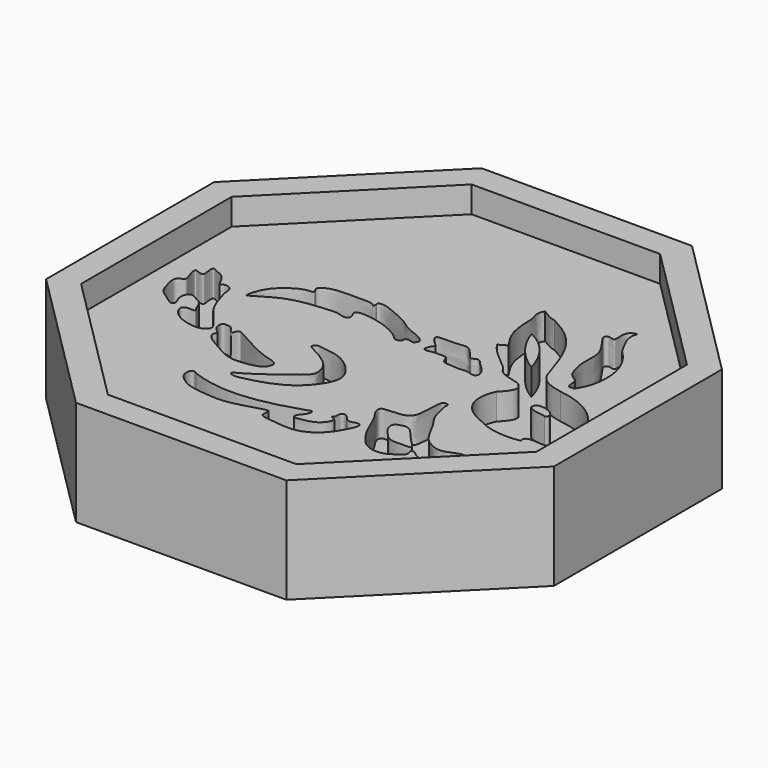
from build123d import *

# Parameters (mm, degrees)
F1_DEPTH = 25.4
F3_DEPTH = 6.35
F5_DEPTH = 6.35


with BuildPart() as f1:
    # F0 (on Top) → F1 (new body)
    with BuildSketch(Plane.XY):
        Polygon((-61.3372846899, 25.3607087968), (-61.3047391097, -25.4392807779), (-25.3607087968, -61.3372846899), (25.4392807779, -61.3047391097), (61.3372846899, -25.3607087968), (61.3047391097, 25.4392807779), (25.3607087968, 61.3372846899), (-25.4392807779, 61.3047391097), align=None)
    extrude(amount=F1_DEPTH)

    # F2 (on face) → F3 (cut)
    with BuildSketch(Plane.XY.offset(25.4)):
        Polygon((-54.9856008905, 22.734521413), (-54.9564255154, -22.8049569991), (-22.734521413, -54.9856008905), (22.8049569991, -54.9564255154), (54.9856008905, -22.734521413), (54.9564255154, 22.8049569991), (22.734521413, 54.9856008905), (-22.8049569991, 54.9564255154), align=None)
    extrude(amount=-F3_DEPTH, mode=Mode.SUBTRACT)

    # F4 (on face) → F5 (cut)
    with BuildSketch(Plane.XY.offset(19.05)):
        with BuildLine():
            add(Edge.make_bspline(
                [(12.8652052954, 32.6095893979), (14.2863783985, 31.7213572562), (15.3522584587, 31.0699865222), (16.5365692228, 30.8923404664)],
                knots=[0, 0, 0, 0, 4.0531292825, 4.0531292825, 4.0531292825, 4.0531292825], degree=3))
            add(Edge.make_bspline(
                [(12.8652052954, 32.6095893979), (11.5624647588, 31.0699865222), (12.8652052954, 29.569859306), (12.8652052954, 28.0499942601)],
                knots=[0, 0, 0, 0, 4.5595951378, 4.5595951378, 4.5595951378, 4.5595951378], degree=3))
            add(Edge.make_bspline(
                [(12.8652052954, 28.0499942601), (12.8652052954, 21.7139329761), (14.3455937505, 20.2335454524), (16.1220598966, 17.450414598)],
                knots=[0, 0, 0, 0, 11.0886514467, 11.0886514467, 11.0886514467, 11.0886514467], degree=3))
            add(Edge.make_bspline(
                [(16.1220598966, 17.450414598), (15.4904279237, 17.0951218655), (14.8587959508, 16.739829133), (14.2271639779, 16.3845364004)],
                knots=[0, 0, 0, 0, 2.1741036945, 2.1741036945, 2.1741036945, 2.1741036945], degree=3))
            add(Edge.make_bspline(
                [(14.2271639779, 16.3845364004), (16.4181385189, 12.7723887563), (20.6816550344, 10.9367063269), (21.8067504466, 8.5088703781)],
                knots=[0, 0, 0, 0, 10.930519033, 10.930519033, 10.930519033, 10.930519033], degree=3))
            add(Edge.make_bspline(
                [(21.8067504466, 8.5088703781), (23.6424319446, 6.8508354016), (27.4914409965, 6.9692670368), (27.6098717004, 5.9626027942)],
                knots=[0, 0, 0, 0, 6.3371677346, 6.3371677346, 6.3371677346, 6.3371677346], degree=3))
            add(Edge.make_bspline(
                [(27.6098717004, 5.9626027942), (28.7349671125, 5.3704483435), (28.9126131684, 3.9492752403), (26.1294841766, 1.2845764868)],
                knots=[0, 0, 0, 0, 4.9066768136, 4.9066768136, 4.9066768136, 4.9066768136], degree=3))
            add(Edge.make_bspline(
                [(26.1294841766, 1.2845764868), (23.7016472965, -4.3408987112), (26.3663455844, -7.9530458897), (31.2812328339, -9.8479427397)],
                knots=[0, 0, 0, 0, 12.2667639806, 12.2667639806, 12.2667639806, 12.2667639806], degree=3))
            add(Edge.make_bspline(
                [(31.2812328339, -9.8479427397), (35.0975431502, -11.920648627), (38.6735312641, -12.0461210608), (41.9044718146, -11.5755964071)],
                knots=[0, 0, 0, 0, 10.7628060299, 10.7628060299, 10.7628060299, 10.7628060299], degree=3))
            add(Edge.make_bspline(
                [(41.9044718146, -11.5755964071), (42.085633815, -11.5042446954), (42.4448295561, -11.3627733554), (41.9699487847, -10.9055818356), (42.4013458456, -10.2892093312), (42.9700330767, -9.9623558206), (44.339317482, -9.9303609692), (45.9999484886, -10.2190009461), (48.2650632898, -10.0226477297), (49.0421733777, -8.4974348176), (49.4673986841, -6.7818760612), (48.2356150706, -6.0112838819), (48.2111816709, -5.1344445173), (48.9546428188, -4.7180950966), (49.1552088222, -4.3385691075), (49.2499768734, -4.1592419147)],
                knots=[0, 0, 0, 0, 0.0517926528, 0.1026909632, 0.163872049, 0.2257582337, 0.3131365022, 0.4162991716, 0.5271779503, 0.6246107168, 0.7212866458, 0.8073521373, 0.8713533909, 0.939214083, 1, 1, 1, 1], degree=3))
            add(Edge.make_bspline(
                [(35.6039665639, 8.8641643524), (44.6259453893, 7.657723967), (49.1314120591, 2.2432615515), (49.2499768734, -4.1592419147)],
                knots=[0, 0, 0, 0, 18.8632634548, 18.8632634548, 18.8632634548, 18.8632634548], degree=3))
            add(Edge.make_bspline(
                [(29.0902592242, 13.4237594903), (29.9192778766, 10.0484741852), (33.2945622504, 9.3378880993), (35.6039665639, 8.8641643524)],
                knots=[0, 0, 0, 0, 7.9509930907, 7.9509930907, 7.9509930907, 7.9509930907], degree=3))
            add(Edge.make_bspline(
                [(16.5365692228, 30.8923404664), (24.7083120048, 26.7472546548), (26.1886995286, 22.1876576543), (29.0902592242, 13.4237594903)],
                knots=[0, 0, 0, 0, 21.5115423429, 21.5115423429, 21.5115423429, 21.5115423429], degree=3))
        make_face()
        with BuildLine():
            add(Edge.make_bspline(
                [(35.1602807641, 0.4698429548), (36.2895391881, -0.722153578), (38.6735312641, -0.5339434138), (39.4263714552, -0.8476267685)],
                knots=[0, 0, 0, 0, 4.4648915168, 4.4648915168, 4.4648915168, 4.4648915168], degree=3))
            add(Edge.make_bspline(
                [(35.1602807641, 0.4698429548), (35.003438592, 1.9127863925), (36.3522768021, 2.069628099), (37.8579571843, 1.6618396621)],
                knots=[0, 0, 0, 0, 2.9492904602, 2.9492904602, 2.9492904602, 2.9492904602], degree=3))
            add(Edge.make_bspline(
                [(37.8579571843, 1.6618396621), (40.5870005488, 0.8148947963), (40.3674244881, -1.0985733243), (39.4263714552, -0.8476267685)],
                knots=[0, 0, 0, 0, 2.9592811782, 2.9592811782, 2.9592811782, 2.9592811782], degree=3))
        make_face(mode=Mode.SUBTRACT)
        with BuildLine():
            add(Edge.make_bspline(
                [(16.5957845747, 23.8456930965), (17.7208781242, 20.1151147485), (20.8000857383, 15.6739503145), (25.0043887645, 13.2461134344)],
                knots=[0, 0, 0, 0, 13.5298083295, 13.5298083295, 13.5298083295, 13.5298083295], degree=3))
            add(Edge.make_bspline(
                [(16.5957845747, 23.8456930965), (21.1553797126, 21.7139348388), (23.8792933524, 17.6280625165), (25.0043887645, 13.2461134344)],
                knots=[0, 0, 0, 0, 13.5298083295, 13.5298083295, 13.5298083295, 13.5298083295], degree=3))
        make_face(mode=Mode.SUBTRACT)
        with BuildLine():
            add(Edge.make_bspline(
                [(36.7773883045, 11.3904932514), (36.5258197984, 11.4134308161), (36.0059714744, 11.441552121), (35.4683105712, 11.2022950388), (35.0849477198, 12.6846305445), (35.2044017719, 13.6366200305), (34.6569395769, 14.4413469981), (33.0252024985, 15.2566678667), (32.1524743097, 17.1164486402), (31.1629146199, 20.9798916279), (32.1715119956, 26.1591358134), (27.9018010841, 30.7101153681), (28.0217561467, 31.6738305022), (28.8396744959, 32.2666284081), (30.5133899031, 31.2777787574), (30.1501733126, 33.751637451), (30.3635645033, 35.1293956273), (31.0534006719, 35.9831194527), (32.5217684997, 36.4324470209), (31.9141483837, 35.4262952592), (31.9752447746, 33.6444442125), (32.6877917851, 32.0781371573), (33.7237389019, 29.9957571139), (34.2604020968, 29.1530700042), (34.501876682, 28.7738982588)],
                knots=[0, 0, 0, 0, 0.0319635023, 0.0550969569, 0.0962347495, 0.1325275562, 0.165994293, 0.2132001677, 0.2639019916, 0.3346772161, 0.4182092739, 0.5039036206, 0.5343069472, 0.567289738, 0.6075861256, 0.6559940549, 0.7003539611, 0.7383866916, 0.7752241506, 0.8051753553, 0.853499607, 0.9018762488, 0.9566720551, 1, 1, 1, 1], degree=3))
            add(Edge.make_bspline(
                [(36.7773883045, 11.3904932514), (39.463236928, 14.7851072252), (40.5450351536, 23.2529882342), (34.501876682, 28.7738982588)],
                knots=[0, 0, 0, 0, 17.5317062146, 17.5317062146, 17.5317062146, 17.5317062146], degree=3))
        make_face()
        with BuildLine():
            add(Edge.make_bspline(
                [(15.3017798439, 4.1850977577), (15.8504108693, 4.2177850474), (16.5550414794, 4.4887049852), (18.1896166173, 3.7142435012), (18.9757283165, 3.942597704), (19.4289979449, 4.7489757975), (18.5062489089, 6.7036354871), (16.5855031627, 8.1069206623), (15.8635662747, 9.3024818194), (14.8371871759, 9.4871226277), (14.006117554, 8.7324291205), (13.103768358, 9.4594760938), (12.3172770418, 10.6148024398), (10.7037012869, 12.421894333), (8.2663371615, 11.8028060837), (4.898617779, 11.9776625169), (2.8500336424, 11.7387445434), (4.0240421234, 10.0496599019), (4.8411169475, 9.3131721564), (5.6861925994, 8.7314147789), (4.8632757263, 7.994538167), (4.123946878, 5.7617188641), (7.0646114832, 6.6737619756), (9.4938960044, 6.3797840159), (10.0551516797, 6.4343790069), (10.5890638145, 4.3108599447), (12.1918688277, 4.4285767471), (14.4613292593, 4.1350239368), (15.3017798439, 4.1850977577)],
                knots=[0, 0, 0, 0, 0.0361277896, 0.0763539638, 0.1028571999, 0.1295711882, 0.1739091507, 0.2230620953, 0.2589689593, 0.2882258976, 0.3185345855, 0.3486027423, 0.3867925471, 0.4326179474, 0.4806856441, 0.5402453162, 0.5771081861, 0.6152551567, 0.6508315792, 0.6775455624, 0.7080799002, 0.7471334048, 0.7948687597, 0.8449259197, 0.8652135961, 0.9066525536, 0.9446556602, 1, 1, 1, 1], degree=3))
        make_face()
        with BuildLine():
            add(Edge.make_bspline(
                [(20.7343194634, -10.3275906295), (20.7709516831, -9.8598877606), (20.9158013429, -9.1476544453), (20.9635707176, -8.3262617691), (22.6524519262, -8.4637543763), (22.1858573154, -9.2863129669), (22.8103442257, -11.5488357773), (23.5016327468, -14.4918837995), (25.2439746955, -16.479295255), (26.7192648498, -19.6806321358), (28.4820205578, -22.3893117533), (30.5649842324, -23.6079937955), (32.7224685673, -24.3807567966), (35.2730051603, -23.378210488), (37.5654236583, -22.4783010118), (39.5446386208, -23.2424793874), (40.5050746182, -24.7881204138), (39.5650007167, -26.4962867217), (37.8128469366, -27.376918268), (35.2912661081, -28.2581182564), (33.3702752918, -28.9782017348), (30.9937489589, -29.088417311), (29.8397340381, -27.8310551705), (29.2156467184, -27.5106948573), (28.5387591084, -27.5359211724), (28.9890389277, -28.7818359483), (28.8075987021, -29.5377697234), (27.5485780868, -30.3867738592), (25.8135024785, -31.7677621319), (22.9716312634, -32.1429236281), (20.6399509233, -31.1555623423), (19.1403603495, -29.7183893954), (17.218559592, -26.9586403206), (16.1693959068, -24.4259222885), (14.8228571758, -21.2324016074), (13.1046488012, -19.1566371774), (13.2906663008, -17.6254241158), (14.4140267208, -17.4507651836), (16.5397677874, -17.2745262674), (18.8545261878, -17.2235756021), (20.4165119591, -15.7458789134), (20.4603473095, -14.0004061218), (20.7425460097, -12.1928979064), (20.6897030651, -10.8972317167), (20.7343194634, -10.3275906295)],
                knots=[0, 0, 0, 0, 0.0192942462, 0.0330741582, 0.052023046, 0.0651534831, 0.0913607937, 0.1216682951, 0.1495277699, 0.1820289015, 0.2130205143, 0.2394568776, 0.2648206079, 0.2930684248, 0.3200314682, 0.3440938321, 0.3657476976, 0.3880714073, 0.4123425116, 0.4405060774, 0.4657585875, 0.4915198065, 0.5133109298, 0.5277187881, 0.5387754002, 0.5568241908, 0.5717634667, 0.5922524986, 0.6181648002, 0.6469137153, 0.6737437891, 0.6986364849, 0.7298941842, 0.7590226893, 0.7913338923, 0.8195504419, 0.8381811992, 0.8549448831, 0.8804793546, 0.9068513478, 0.9306238126, 0.9529472238, 0.9765004747, 1, 1, 1, 1], degree=3))
        make_face()
        with BuildLine():
            add(Edge.make_bspline(
                [(22.8049569991, -26.4832917601), (21.7773803974, -26.1427349942), (20.7853597636, -24.7888072098), (19.4526932441, -23.4275348596), (19.0202822949, -21.3443208318), (20.4823026858, -20.6843131009), (22.5005362497, -20.2861010048), (24.4630261175, -22.5402330727), (26.0115860218, -24.4108868337), (27.5192963017, -25.7368526878), (27.8767415454, -26.6402760759), (27.0016791884, -26.6409491135), (24.1151934487, -26.917526918), (22.8049569991, -26.4832917601)],
                knots=[0, 0, 0, 0, 0.1074165587, 0.1986974636, 0.2853810353, 0.3613910674, 0.4510317064, 0.5602063852, 0.6661241164, 0.759241241, 0.8125419066, 0.8630359136, 1, 1, 1, 1], degree=3))
        make_face(mode=Mode.SUBTRACT)
        with BuildLine():
            add(Edge.make_bspline(
                [(-22.8500030935, -28.2156076282), (-23.1564221999, -28.0159332998), (-23.7152769634, -27.6517623089), (-24.3863424084, -28.1871627376), (-24.5625231079, -29.9486699359), (-23.3433241377, -31.3252949477), (-20.9932031236, -33.2067386928), (-15.22638086, -33.8351646845), (-10.1785100814, -34.0688360581), (-2.47913326, -31.1920867638), (-2.460426325, -32.046776882), (-2.3970225018, -32.8404748019), (-2.810640208, -34.2142542547), (2.0819787419, -34.5708039142), (6.7193859797, -35.1778319566), (11.7912536807, -32.1183129725), (14.0526674831, -27.6010297002), (14.5257017357, -26.4335554129), (14.6297205539, -25.2558639264), (13.4476452439, -25.0434674258), (12.677210255, -25.5824518196), (11.8921264481, -25.5053919057), (11.1659879121, -25.3350906316), (10.7521041426, -24.4270564162), (9.6833422485, -23.7478146611), (8.9110694031, -23.9254162985), (8.6366931415, -24.8331893315), (8.8904588509, -25.5996048999), (7.9621028526, -26.2811431455), (9.3608334823, -26.3303129622), (9.4999519076, -27.552032903), (7.796632177, -29.9619376165), (4.804334332, -30.4744649523), (3.3250515889, -30.808696151), (2.4506336317, -30.5166183135), (2.6073700045, -29.6227983207), (3.5136911361, -28.6934956319), (4.0114212731, -27.9436231109), (4.2838183347, -26.8876544187), (3.8082859259, -26.5723866906), (3.3697701718, -26.7870327785), (3.1157024205, -26.9113946706)],
                knots=[0, 0, 0, 0, 0.0200132257, 0.0365006172, 0.0622847867, 0.0892370717, 0.124007682, 0.1718500922, 0.2222414582, 0.2769290002, 0.2891044901, 0.3077607047, 0.3273219132, 0.3688671667, 0.4147463647, 0.4634655653, 0.5085506795, 0.5315635247, 0.5511247333, 0.5709731652, 0.5906705705, 0.6084161703, 0.6252452309, 0.6452755692, 0.6677696463, 0.6843028154, 0.7030430888, 0.721261059, 0.7378696831, 0.75676453, 0.7765156316, 0.8105318006, 0.8462195329, 0.8714235324, 0.888436846, 0.9057622096, 0.9290789036, 0.9493112706, 0.9693926854, 0.9822666996, 1, 1, 1, 1], degree=3))
            add(Edge.make_bspline(
                [(3.1157024205, -26.9113946706), (-6.5275733359, -30.1126465201), (-14.4714191556, -31.4168594778), (-22.8500030935, -28.2156076282)],
                knots=[0, 0, 0, 0, 25.9984390738, 25.9984390738, 25.9984390738, 25.9984390738], degree=3))
        make_face()
        with BuildLine():
            add(Edge.make_bspline(
                [(-10.6559619308, -5.2117551677), (-11.1737401757, -5.1362324872), (-11.7424506379, -4.9714464397), (-12.648442391, -5.4144357157), (-12.7500393741, -6.1161411911), (-12.3125446671, -6.4565452867), (-10.9405308104, -7.0731225678), (-9.1369698619, -8.0823065363), (-6.0712570972, -10.2151958876), (-5.2217867694, -12.6447334736), (-4.9746455567, -14.6813205825), (-7.5588855144, -16.9055478606), (-10.6532169743, -19.0485081325), (-14.4504219336, -22.0939945512), (-17.455448897, -23.5012935564), (-17.9230491301, -24.1027794323), (-16.6706066398, -24.7404310598), (-13.7255998954, -24.156814816), (-5.3862465252, -21.8767233991), (0.0120330444, -15.0338509057), (-0.1770248658, -10.6283446412), (-5.2708543932, -5.5843953024), (-9.5773732915, -5.3690771603), (-10.6559619308, -5.2117551677)],
                knots=[0, 0, 0, 0, 0.0310574833, 0.0576453165, 0.0794112577, 0.0992654413, 0.1335769874, 0.1762031417, 0.2313178012, 0.276910693, 0.3154710571, 0.3660978136, 0.4233404628, 0.4884366707, 0.5399210219, 0.5589256006, 0.5872706354, 0.636270169, 0.7212275866, 0.803887594, 0.8604004895, 0.9353038701, 1, 1, 1, 1], degree=3))
        make_face()
        with BuildLine():
            add(Edge.make_bspline(
                [(-22.2946368158, -19.1632434726), (-21.0493988148, -19.5119202164), (-18.6880382006, -19.4450553681), (-15.5481418092, -18.8919910447), (-14.0332293864, -17.8840870443), (-13.4955697372, -16.3469941527), (-14.1341895958, -15.4339327932), (-16.3883421895, -14.9050941461), (-19.8490922568, -13.5739760108), (-22.5931502921, -11.9756349915), (-26.078519987, -10.2568666189), (-26.8991210249, -9.5874929089), (-27.6901522691, -10.13266369), (-27.6203290749, -11.0788339927), (-28.6319524294, -10.7883304604), (-29.308762912, -9.2806269758), (-30.2719479537, -9.3408028948), (-31.8815711607, -8.945568532), (-31.7053750515, -11.3414838731), (-30.60133097, -12.272673542), (-29.7599805353, -12.7489968005), (-30.6848565625, -13.6607693821), (-29.5836041778, -15.4675565989), (-26.3586662834, -17.1279574729), (-23.6842152669, -18.7741502316), (-22.2946368158, -19.1632434726)],
                knots=[0, 0, 0, 0, 0.0622592495, 0.1194842442, 0.1621790015, 0.2007002522, 0.2312415619, 0.2794627383, 0.3419096516, 0.4020814388, 0.4652367387, 0.4959773841, 0.5239430148, 0.5511816552, 0.578209774, 0.6183631416, 0.649465769, 0.6848743271, 0.7281984959, 0.7682926938, 0.7951052662, 0.8255927665, 0.8680347902, 0.9305240353, 1, 1, 1, 1], degree=3))
        make_face()
        with BuildLine():
            add(Edge.make_bspline(
                [(-48.536233604, 0.5818881327), (-48.7993935081, 0.214424348), (-50.6232341136, -0.1406925801), (-49.5900537739, -3.567871753), (-48.9612726452, -6.0753250269), (-45.8419759594, -7.8890615195), (-44.5461860731, -8.9553314596), (-43.668018572, -8.2975634323), (-44.3455154017, -7.0124013614), (-44.7212608191, -5.7619723643), (-44.5464307201, -4.3277114714), (-43.475906841, -3.4658299441), (-41.9919242331, -4.3530284656), (-40.0910014917, -5.3334169649), (-39.7171833038, -7.116003175), (-38.6376000967, -8.4834991304), (-40.0099629337, -8.3881716907), (-41.220260459, -8.31457224), (-41.9367437761, -9.1059292531), (-41.7226121814, -9.6941307646), (-41.4943253777, -10.5163335894), (-39.6311525311, -12.4424849476), (-36.8731140753, -13.275454031), (-34.5043187855, -13.6223348002), (-32.8528768601, -13.1099659491), (-31.946682489, -12.1411358408), (-32.4510768522, -10.7397642295), (-34.6480914317, -8.2150297923), (-36.3991290059, -6.2732019618), (-37.8806992705, -3.4304789411), (-38.7339927463, -0.5836219813), (-39.1752539851, 1.0003629302), (-39.0635096274, 2.2340517971), (-40.1593292268, 3.6055012549), (-41.8496236937, 3.2097039443), (-41.8184773397, 2.3568461735), (-42.9403272041, 4.6014895605), (-44.0708022394, 6.1878150156), (-45.8347779568, 6.6928819631), (-47.3484563418, 7.7686503404), (-47.0497576663, 5.1475346558), (-46.7874060186, 3.9082822982), (-48.2830523519, 4.2933827218), (-49.6768094639, 4.9815397707), (-48.8456887547, 2.2143254407), (-48.2702506616, 0.9532938716), (-48.536233604, 0.5818881327)],
                knots=[0, 0, 0, 0, 0.0232700879, 0.0539157394, 0.0832957416, 0.1165416169, 0.138415086, 0.1530447808, 0.1731834999, 0.1941072535, 0.214856042, 0.2333825675, 0.2557602784, 0.2813606968, 0.3057129626, 0.3251805072, 0.3419299519, 0.3622670956, 0.3788760639, 0.3918609072, 0.4078158578, 0.4361664442, 0.4668508531, 0.4942472654, 0.5171620156, 0.5358189465, 0.5559576611, 0.5884303759, 0.6178091555, 0.6495379489, 0.6803811716, 0.7028030609, 0.7220480786, 0.7441492982, 0.7654682675, 0.7754510114, 0.7999460146, 0.8261963933, 0.8505486575, 0.8693192598, 0.8947421061, 0.9124104213, 0.9322578942, 0.9497491424, 0.9764802831, 1, 1, 1, 1], degree=3))
        make_face()
        with BuildLine():
            add(Edge.make_bspline(
                [(-14.9078318116, 9.9650415808), (-14.5439237612, 10.543552861), (-10.1816380527, 10.1455622924), (-6.735553481, 9.0283916293), (-3.5389546047, 7.4079014565), (-2.2665814543, 5.884788011), (-1.5730472986, 6.1126504048), (-0.7286873877, 6.2004641081), (-0.8992384984, 7.3134721768), (0.020145302, 7.6483964059), (1.2671100812, 6.9765688977), (1.6396581827, 7.5405290547), (2.0943183966, 8.2303649287), (1.3649219897, 9.2347624028), (-0.9541283771, 10.3285701067), (-3.3477979505, 11.084743311), (-5.2206670384, 12.7962188062), (-8.6746986904, 14.3125128641), (-12.7872399151, 16.1392624124), (-14.2109690291, 15.3069253956), (-13.6726261286, 15.1739510755), (-13.9056025795, 13.8580480834), (-14.2641332952, 14.9144076807), (-17.6290630724, 14.9469588147), (-20.7581041002, 14.9579080496), (-25.0931402223, 14.7764746628), (-26.9152070911, 13.0760185626), (-26.5534669737, 12.4622646115), (-25.8655118726, 11.3650312617), (-27.815335632, 11.4557675225), (-30.3612376481, 10.4162226176), (-34.2377667405, 7.2671161354), (-35.2268045131, 3.6505780257), (-35.5300227841, 2.2890931816), (-33.9755773185, 3.2390069932), (-32.9625297054, 3.7546067761), (-29.0387096882, 6.3511254429), (-23.4106114174, 7.3179662907), (-20.1678580514, 7.566163094), (-17.2711363372, 7.8301236671), (-15.8324958608, 7.0635253095), (-14.4759035427, 7.2167301906), (-14.2916378146, 8.4286175303), (-15.1329919604, 9.6071003763), (-14.9078318116, 9.9650415808)],
                knots=[0, 0, 0, 0, 0.0353575458, 0.0709401714, 0.1032054593, 0.1259091647, 0.139493691, 0.1536451156, 0.1696227785, 0.1848328811, 0.2041888568, 0.2167714454, 0.231345754, 0.2487436603, 0.2763912348, 0.3037690537, 0.3304351456, 0.3647331065, 0.4013398346, 0.4183208749, 0.4274962573, 0.4437526218, 0.4555748073, 0.4857968801, 0.5182328685, 0.5540044498, 0.5784209693, 0.5917937196, 0.6077288292, 0.6275338448, 0.6567676036, 0.695218605, 0.7287351036, 0.7436854924, 0.7630890438, 0.7826676884, 0.81914689, 0.8608357338, 0.8923502694, 0.920908852, 0.942706714, 0.9606601027, 0.9781232917, 1, 1, 1, 1], degree=3))
        make_face()
    extrude(amount=-F5_DEPTH, mode=Mode.SUBTRACT)


solid = f1.part
